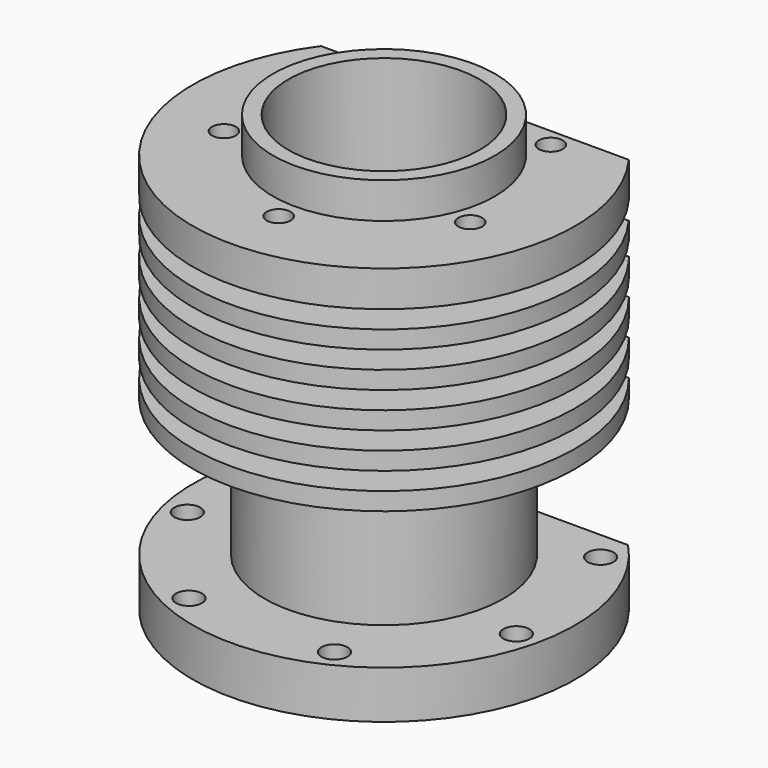
from build123d import *

# Parameters (mm, degrees)
F0_R      = 25.4
F1_DEPTH  = 53.0098
F2_R      = 14.732
F3_DEPTH  = 4.7625
F4_R      = 15.875
F5_DEPTH  = 3.175
F7_R      = 12.7
F8_DEPTH  = 60.9483
F9_W      = 12.1422023922
F9_H      = 2.3622
F11_W     = 13.3322854936
F11_H     = 18.2753
F14_DEPTH = 11.8618
F16_DEPTH = 16.637
F18_DEPTH = 6.477
F20_D     = 3.4544
F20_DEPTH = 7.62
F20_TIP   = 1.0378064612
F22_D     = 3.175
F22_DEPTH = 6.35
F22_TIP   = 0.9538662327


# Not quite as in the source:
# - a feature names something its author has since deleted; it is built from what else it names


with BuildPart() as f1:
    # F0 (on Top) → F1 (new body)
    with BuildSketch(Plane.XY):
        Circle(F0_R)
    extrude(amount=F1_DEPTH)

    # F2 (on face) → F3 (join)
    with BuildSketch(Plane.XY.offset(53.0098)):
        Circle(F2_R)
    extrude(amount=F3_DEPTH)

    # F4 (on face) → F5 (join)
    with BuildSketch(Plane(origin=(0, 0, 0), x_dir=(1, 0, 0), z_dir=(0, 0, -1))):
        Circle(F4_R)
    extrude(amount=F5_DEPTH)

    # F7 (on face) → F8 (cut, through all)
    with BuildSketch(Plane(origin=(0, 0, -3.175), x_dir=(1, 0, 0), z_dir=(0, 0, -1))):
        Circle(F7_R)
    extrude(amount=-F8_DEPTH, mode=Mode.SUBTRACT)

    # F9 (on Front) → F10 (revolve, cut)
    with BuildSketch(Plane.XZ):
        with Locations((21.9461011961, 47.0662)):
            Rectangle(F9_W, F9_H)
        with Locations((21.9461011961, 42.3418)):
            Rectangle(F9_W, F9_H)
        with Locations((21.9461011961, 37.6174)):
            Rectangle(F9_W, F9_H)
        with Locations((21.9461011961, 32.893)):
            Rectangle(F9_W, F9_H)
        with Locations((21.9461011961, 28.1686)):
            Rectangle(F9_W, F9_H)
    revolve(axis=Axis((0, 0, 0), (0, 0, -1)), mode=Mode.SUBTRACT)

    # F11 (on Front) → F12 (revolve, cut)
    with BuildSketch(Plane.XZ):
        with Locations((22.5411427468, 15.48765)):
            Rectangle(F11_W, F11_H)
    revolve(axis=Axis((0, 0, 0), (0, 0, -1)), mode=Mode.SUBTRACT)

    # F13 (on face) → F14 (cut)
    with BuildSketch(Plane.XY.offset(53.0098)):
        with BuildLine():
            Line((-28.8578128478, 32.0924090841), (-28.8578128478, 15.0876))
            Line((-28.8578128478, 15.0876), (-20.4334120068, 15.0876))
            ThreePointArc((-20.4334120068, 15.0876), (0, 25.4), (20.4334120068, 15.0876))
            Line((20.4334120068, 15.0876), (35.4937171599, 15.0876))
            Line((35.4937171599, 15.0876), (35.4937171599, 32.0924090841))
            Line((35.4937171599, 32.0924090841), (-28.8578128478, 32.0924090841))
        make_face()
        with BuildLine():
            ThreePointArc((20.4334120068, 15.0876), (0, 25.4), (-20.4334120068, 15.0876))
            Line((-20.4334120068, 15.0876), (20.4334120068, 15.0876))
        make_face()
    extrude(amount=-F14_DEPTH, mode=Mode.SUBTRACT)

    # F15 (on face) → F16 (cut)
    with BuildSketch(Plane.XY.offset(41.148)):
        with BuildLine():
            Line((22.7077871409, 25.7988459408), (-23.4762642381, 25.7988459408))
            Line((-23.4762642381, 25.7988459408), (-23.4762642381, 15.875))
            Line((-23.4762642381, 15.875), (-19.8278686449, 15.875))
            ThreePointArc((-19.8278686449, 15.875), (0, 25.4), (19.8278686449, 15.875))
            Line((19.8278686449, 15.875), (22.7077871409, 15.875))
            Line((22.7077871409, 15.875), (22.7077871409, 25.7988459408))
        make_face()
        with BuildLine():
            ThreePointArc((19.8278686449, 15.875), (0, 25.4), (-19.8278686449, 15.875))
            Line((-19.8278686449, 15.875), (19.8278686449, 15.875))
        make_face()
    extrude(amount=-F16_DEPTH, mode=Mode.SUBTRACT)

    # F17 (on face) → F18 (cut)
    with BuildSketch(Plane(origin=(0, 0, 0), x_dir=(1, 0, 0), z_dir=(0, 0, -1))):
        with BuildLine():
            Line((-18.4330514283, -17.4752), (-34.0658536954, -17.4752))
            Line((-34.0658536954, -17.4752), (-34.0658536954, -39.2576220664))
            Line((-34.0658536954, -39.2576220664), (38.0722320481, -39.2576220664))
            Line((38.0722320481, -39.2576220664), (38.0722320481, -17.4752))
            Line((38.0722320481, -17.4752), (18.4330514283, -17.4752))
            ThreePointArc((18.4330514283, -17.4752), (0, -25.4), (-18.4330514283, -17.4752))
        make_face()
        with BuildLine():
            Line((18.4330514283, -17.4752), (-18.4330514283, -17.4752))
            ThreePointArc((-18.4330514283, -17.4752), (0, -25.4), (18.4330514283, -17.4752))
        make_face()
    extrude(amount=-F18_DEPTH, mode=Mode.SUBTRACT)

    # F20
    with Locations(Plane(origin=(0, 0, 0), x_dir=(1, 0, 0), z_dir=(0, 0, -1))):
        with Locations((-17.907, -13.5636), (-21.844, 5.334), (-9.652, 20.2946), (9.652, 20.2946), (21.844, 5.334), (17.907, -13.5636)):
            Hole(F20_D / 2, depth=F20_DEPTH)
            with Locations((0, 0, -(F20_DEPTH + F20_TIP / 2))):  # 118° drill point
                Cone(0, F20_D / 2, F20_TIP, mode=Mode.SUBTRACT)

    # F22
    with Locations(Plane.XY.offset(53.0098)):
        with Locations((-12.0142, 12.6746), (12.0142, 12.6746), (16.3576, -6.1214), (-16.3576, -6.1214), (0, -17.4752)):
            Hole(F22_D / 2, depth=F22_DEPTH)
            with Locations((0, 0, -(F22_DEPTH + F22_TIP / 2))):  # 118° drill point
                Cone(0, F22_D / 2, F22_TIP, mode=Mode.SUBTRACT)


solid = f1.part
